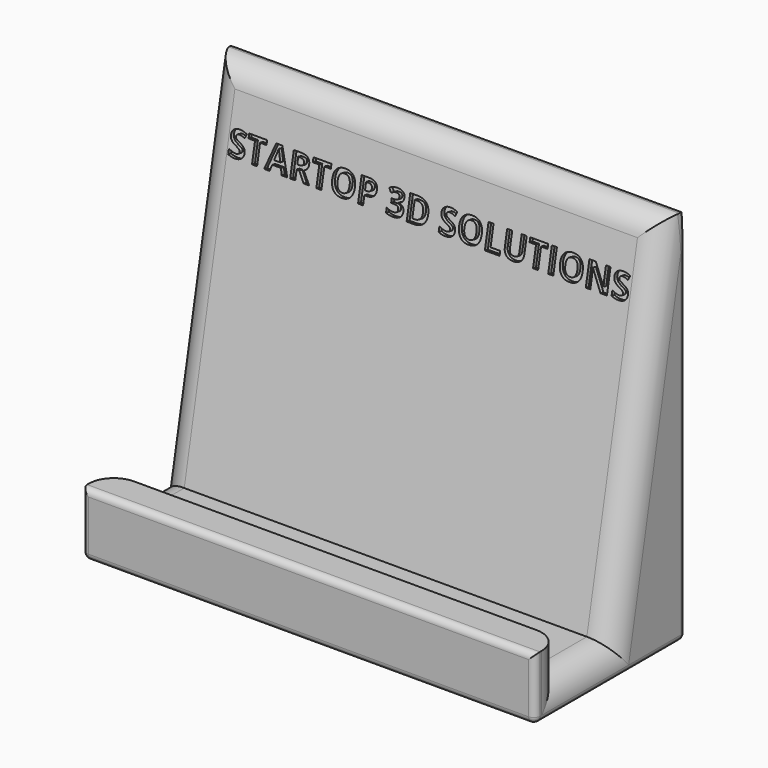
from build123d import *

# Parameters (mm, degrees)
F1_DEPTH     = 91.44
F2_T1_DEPTH  = 112.3781441998
F2_T3_DEPTH  = 19.05
F2_T8_DEPTH  = 96.5573611426
F2_T13_DEPTH = 96.5573611426
F2_T18_DEPTH = 25.4
F2_T23_DEPTH = 25.4
F2_T29_DEPTH = 96.5573611426
F2_T34_DEPTH = 25.4
F2_T41_DEPTH = 96.5573611426
F2_T46_DEPTH = 25.4
F2_T53_DEPTH = 19.05
F2_T58_DEPTH = 38.1
F2_T66_DEPTH = 19.05
F2_T71_DEPTH = 38.1
F3_R         = 1.26999
F4_TEXT_SIZE = 6.73039203
F5_DEPTH     = 0.762


# Not quite as in the source:
# - a fillet or chamfer that OpenCascade refuses, or shapes differently, is made with other operations: its cross-section is extruded or revolved along the edge and cut away or added
# - a fillet or chamfer is up to 0.001 mm smaller than in the source, because OpenCascade refuses the exact size
# - Text() gives the source's letters only with a copy of the font that has no kerning and outlines rounded to 1/6400 em; it was checked with that copy


with BuildPart() as f1:
    # F0 (on Right) → F1 (new body)
    with BuildSketch(Plane.YZ):
        Polygon((0, 12.7), (0, 0), (38.1, 0), (38.1, 76.2), (33.02, 76.2), (19.4425354067, 6.35), (6.7425354067, 6.35), (6.7425354067, 12.7), align=None)
    extrude(amount=F1_DEPTH)

    # F2: fillet of radius 5.08 on 7 edges, made by hand

    # F2_s2 → F2_t1 (cut)
    with BuildSketch(Plane.YZ.offset(-10.4690720999)):
        with BuildLine():
            ThreePointArc((37.20762884, 76.2), (33.9763514809, 75.0398528836), (32.220962748, 72.0893096965))
            Line((32.220962748, 72.0893096965), (33.02, 76.2))
            Line((33.02, 76.2), (37.20762884, 76.2))
        make_face()
    extrude(amount=F2_T1_DEPTH, mode=Mode.SUBTRACT)

    # F2_s4 → F2_t3 (cut)
    with BuildSketch(Plane.XY.offset(6.35)):
        with BuildLine():
            ThreePointArc((5.08, 6.7425354067), (1.4878975516, 5.2546378552), (0, 1.6625354067))
            Line((0, 1.6625354067), (0, 6.7425354067))
            Line((0, 6.7425354067), (5.08, 6.7425354067))
        make_face()
        with BuildLine():
            ThreePointArc((86.36, 6.7425354067), (89.9521024484, 5.2546378552), (91.44, 1.6625354067))
            Line((91.44, 1.6625354067), (91.44, 6.7425354067))
            Line((91.44, 6.7425354067), (86.36, 6.7425354067))
        make_face()
    extrude(amount=F2_T3_DEPTH, mode=Mode.SUBTRACT)


with BuildPart() as f2_tool6:
    # F2_s7 → F2_t8 (new body)
    with BuildSketch(Plane(origin=(0, 17.8979800115, 92.0771249461), x_dir=(1, 0, 0), z_dir=(0, -0.1908089954, -0.9816271834))):
        with BuildLine():
            ThreePointArc((86.36, -17.8736841497), (89.9521024484, -19.3615817013), (91.44, -22.9536841497))
            Line((91.44, -22.9536841497), (91.44, -17.8736841497))
            Line((91.44, -17.8736841497), (86.36, -17.8736841497))
        make_face()
    extrude(amount=F2_T8_DEPTH)

    split(bisect_by=Plane.XY.offset(6.35), keep=Keep.TOP)


with BuildPart() as f1_1:
    add(f1.part)

    # F2_t5: cut F2_tool6
    add(f2_tool6.part, mode=Mode.SUBTRACT)


with BuildPart() as f2_tool11:
    # F2_s12 → F2_t13 (new body)
    with BuildSketch(Plane(origin=(0, 17.8979800115, 92.0771249461), x_dir=(1, 0, 0), z_dir=(0, -0.1908089954, -0.9816271834))):
        with BuildLine():
            ThreePointArc((5.08, -17.8736841497), (1.4878975516, -19.3615817013), (0, -22.9536841497))
            Line((0, -22.9536841497), (0, -17.8736841497))
            Line((0, -17.8736841497), (5.08, -17.8736841497))
        make_face()
    extrude(amount=F2_T13_DEPTH)

    split(bisect_by=Plane.XY.offset(6.35), keep=Keep.TOP)


with BuildPart() as f1_2:
    add(f1_1.part)

    # F2_t10: cut F2_tool11
    add(f2_tool11.part, mode=Mode.SUBTRACT)


with BuildPart() as f2_tool16:
    # F2_s17 → F2_t18 (new body)
    with BuildSketch(Plane.XZ.offset(-32.1425354067)):
        with BuildLine():
            ThreePointArc((86.36, 6.35), (89.9521024484, 4.8621024484), (91.44, 1.27))
            Line((91.44, 1.27), (91.44, 6.35))
            Line((91.44, 6.35), (86.36, 6.35))
        make_face()
    extrude(amount=F2_T18_DEPTH)

    split(bisect_by=Plane(origin=(0, 17.5452942298, -3.4104597163), x_dir=(1, 0, 0), z_dir=(0, -0.9816271834, 0.1908089954)), keep=Keep.TOP)


with BuildPart() as f1_3:
    add(f1_2.part)

    # F2_t15: cut F2_tool16
    add(f2_tool16.part, mode=Mode.SUBTRACT)


with BuildPart() as f2_tool21:
    # F2_s22 → F2_t23 (new body)
    with BuildSketch(Plane.XZ.offset(-32.1425354067)):
        with BuildLine():
            ThreePointArc((5.08, 6.35), (1.4878975516, 4.8621024484), (0, 1.27))
            Line((0, 1.27), (0, 6.35))
            Line((0, 6.35), (5.08, 6.35))
        make_face()
    extrude(amount=F2_T23_DEPTH)

    split(bisect_by=Plane(origin=(0, 17.5452942298, -3.4104597163), x_dir=(1, 0, 0), z_dir=(0, -0.9816271834, 0.1908089954)), keep=Keep.TOP)


with BuildPart() as f1_4:
    add(f1_3.part)

    # F2_t20: cut F2_tool21
    add(f2_tool21.part, mode=Mode.SUBTRACT)


with BuildPart() as f2_tool27:
    # F2_s28 → F2_t29 (new body)
    with BuildSketch(Plane(origin=(0, 17.8979800115, 92.0771249461), x_dir=(1, 0, 0), z_dir=(0, -0.1908089954, -0.9816271834))):
        with BuildLine():
            ThreePointArc((86.36, -17.8736841497), (89.9521024484, -19.3615817013), (91.44, -22.9536841497))
            Line((91.44, -22.9536841497), (91.44, -17.8736841497))
            Line((91.44, -17.8736841497), (86.36, -17.8736841497))
        make_face()
    extrude(amount=F2_T29_DEPTH)

    split(bisect_by=Plane.XY, keep=Keep.TOP)

    split(bisect_by=Plane.XY.offset(6.35), keep=Keep.BOTTOM)


with BuildPart() as f2_tool32:
    # F2_s33 → F2_t34 (new body)
    with BuildSketch(Plane.XZ.offset(-32.1425354067)):
        with BuildLine():
            ThreePointArc((86.36, 6.35), (89.9521024484, 4.8621024484), (91.44, 1.27))
            Line((91.44, 1.27), (91.44, 6.35))
            Line((91.44, 6.35), (86.36, 6.35))
        make_face()
    extrude(amount=F2_T34_DEPTH)

    split(bisect_by=Plane(origin=(0, 17.5452942298, -3.4104597163), x_dir=(1, 0, 0), z_dir=(0, 0.9816271834, -0.1908089954)), keep=Keep.TOP)


with BuildPart() as f2_tool27_1:
    add(f2_tool27.part)

    # F2_t36: intersect F2_tool32
    add(f2_tool32.part, mode=Mode.INTERSECT)


with BuildPart() as f1_5:
    add(f1_4.part)

    # F2_t25: cut F2_tool27
    add(f2_tool27_1.part, mode=Mode.SUBTRACT)


with BuildPart() as f2_tool39:
    # F2_s40 → F2_t41 (new body)
    with BuildSketch(Plane(origin=(0, 17.8979800115, 92.0771249461), x_dir=(1, 0, 0), z_dir=(0, -0.1908089954, -0.9816271834))):
        with BuildLine():
            ThreePointArc((5.08, -17.8736841497), (1.4878975516, -19.3615817013), (0, -22.9536841497))
            Line((0, -22.9536841497), (0, -17.8736841497))
            Line((0, -17.8736841497), (5.08, -17.8736841497))
        make_face()
    extrude(amount=F2_T41_DEPTH)

    split(bisect_by=Plane.XY, keep=Keep.TOP)

    split(bisect_by=Plane.XY.offset(6.35), keep=Keep.BOTTOM)


with BuildPart() as f2_tool44:
    # F2_s45 → F2_t46 (new body)
    with BuildSketch(Plane.XZ.offset(-32.1425354067)):
        with BuildLine():
            ThreePointArc((5.08, 6.35), (1.4878975516, 4.8621024484), (0, 1.27))
            Line((0, 1.27), (0, 6.35))
            Line((0, 6.35), (5.08, 6.35))
        make_face()
    extrude(amount=F2_T46_DEPTH)

    split(bisect_by=Plane(origin=(0, 17.5452942298, -3.4104597163), x_dir=(1, 0, 0), z_dir=(0, 0.9816271834, -0.1908089954)), keep=Keep.TOP)


with BuildPart() as f2_tool39_1:
    add(f2_tool39.part)

    # F2_t48: intersect F2_tool44
    add(f2_tool44.part, mode=Mode.INTERSECT)


with BuildPart() as f1_6:
    add(f1_5.part)

    # F2_t37: cut F2_tool39
    add(f2_tool39_1.part, mode=Mode.SUBTRACT)


with BuildPart() as f2_tool51:
    # F2_s52 → F2_t53 (new body)
    with BuildSketch(Plane.XY.offset(-6.35)):
        with BuildLine():
            ThreePointArc((86.36, 6.7425354067), (89.9521024484, 5.2546378552), (91.44, 1.6625354067))
            Line((91.44, 1.6625354067), (91.44, 6.7425354067))
            Line((91.44, 6.7425354067), (86.36, 6.7425354067))
        make_face()
    extrude(amount=F2_T53_DEPTH)

    split(bisect_by=Plane.XY, keep=Keep.TOP)

    split(bisect_by=Plane.XY.offset(6.35), keep=Keep.BOTTOM)


with BuildPart() as f2_tool56:
    # F2_s57 → F2_t58 (new body)
    with BuildSketch(Plane.XZ.offset(-32.1425354067)):
        with BuildLine():
            ThreePointArc((86.36, 6.35), (89.9521024484, 4.8621024484), (91.44, 1.27))
            Line((91.44, 1.27), (91.44, 6.35))
            Line((91.44, 6.35), (86.36, 6.35))
        make_face()
    extrude(amount=F2_T58_DEPTH)

    split(bisect_by=Plane.XZ.offset(-6.7425354067), keep=Keep.TOP)

    split(bisect_by=Plane.XZ, keep=Keep.BOTTOM)


with BuildPart() as f2_tool51_1:
    add(f2_tool51.part)

    # F2_t61: intersect F2_tool56
    add(f2_tool56.part, mode=Mode.INTERSECT)


with BuildPart() as f1_7:
    add(f1_6.part)

    # F2_t49: cut F2_tool51
    add(f2_tool51_1.part, mode=Mode.SUBTRACT)


with BuildPart() as f2_tool64:
    # F2_s65 → F2_t66 (new body)
    with BuildSketch(Plane.XY.offset(-6.35)):
        with BuildLine():
            ThreePointArc((5.08, 6.7425354067), (1.4878975516, 5.2546378552), (0, 1.6625354067))
            Line((0, 1.6625354067), (0, 6.7425354067))
            Line((0, 6.7425354067), (5.08, 6.7425354067))
        make_face()
    extrude(amount=F2_T66_DEPTH)

    split(bisect_by=Plane.XY, keep=Keep.TOP)

    split(bisect_by=Plane.XY.offset(6.35), keep=Keep.BOTTOM)


with BuildPart() as f2_tool69:
    # F2_s70 → F2_t71 (new body)
    with BuildSketch(Plane.XZ.offset(-32.1425354067)):
        with BuildLine():
            ThreePointArc((5.08, 6.35), (1.4878975516, 4.8621024484), (0, 1.27))
            Line((0, 1.27), (0, 6.35))
            Line((0, 6.35), (5.08, 6.35))
        make_face()
    extrude(amount=F2_T71_DEPTH)

    split(bisect_by=Plane.XZ.offset(-6.7425354067), keep=Keep.TOP)

    split(bisect_by=Plane.XZ, keep=Keep.BOTTOM)


with BuildPart() as f2_tool64_1:
    add(f2_tool64.part)

    # F2_t74: intersect F2_tool69
    add(f2_tool69.part, mode=Mode.INTERSECT)


with BuildPart() as f1_8:
    add(f1_7.part)

    # F2_t62: cut F2_tool64
    add(f2_tool64_1.part, mode=Mode.SUBTRACT)

    # F3 (radius 1.27 in the source; OpenCascade refuses exactly that, so slightly less here)
    f3_edges = [f1_8.edges().sort_by_distance(p)[0] for p in [
        (0, 38.1, 37.855426),
        (45.72, 38.1, 0),
        (0, 19.05, 0),
        (91.44, 38.1, 37.855426),
        (91.44, 19.05, 0),
        (91.44, 0, 6.35),
        (45.72, 0, 12.7),
        (45.72, 0, 0),
        (0, 0, 6.35),
        (45.72, 38.1, 76.2),
    ]]
    fillet(f3_edges, radius=F3_R)

    # F4 (on face) → F5 (cut)
    with BuildSketch(Plane(origin=(0, 17.5452942298, -3.4104597163), x_dir=(1, 0, 0), z_dir=(0, -0.9816271834, 0.1908089954))):
        with Locations((5.08, 65.8231432634)):
            Text('STARTOP 3D SOLUTIONS', F4_TEXT_SIZE, font='Open Sans', font_style=FontStyle.BOLD, text_align=(TextAlign.LEFT, TextAlign.BOTTOM))
    extrude(amount=-F5_DEPTH, mode=Mode.SUBTRACT)


solid = f1_8.part
